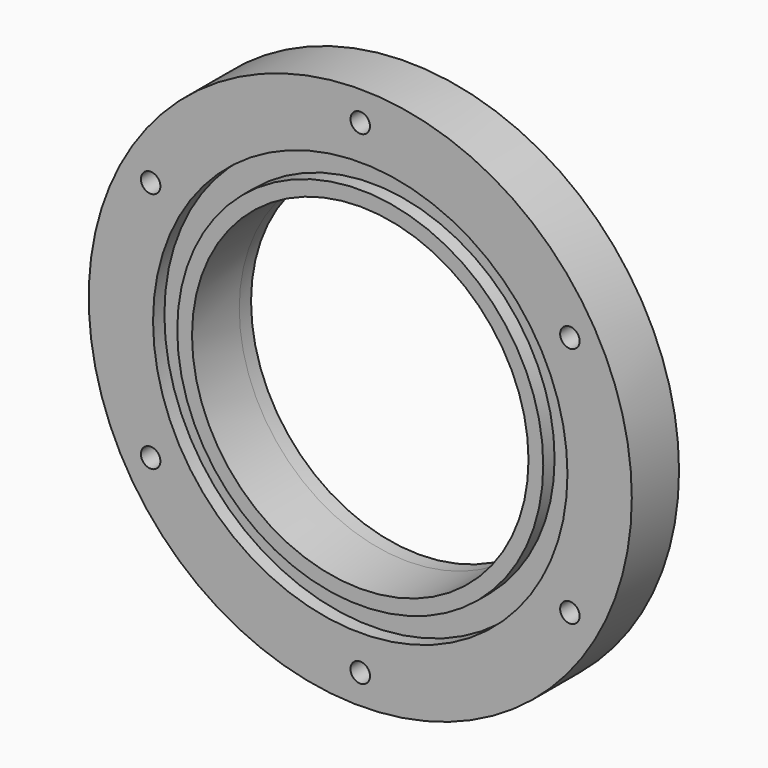
from build123d import *
from build123d import SkipClean  # not in build123d's __all__

# Parameters (mm, degrees)
F0_R     = 46
F0_R_2   = 28.5
F1_DEPTH = 10
F2_R     = 35.1
F2_R_2   = 31
F3_DEPTH = 2.4
F5_D     = 3.3
F5_DEPTH = 8
F5_TIP   = 0.9914200214
F6_R     = 30.5
F6_R_2   = 28.5
F7_DEPTH = 2.5


with BuildPart() as f1:
    # F0 (on Front) → F1 (new body)
    with BuildSketch(Plane.XZ):
        Circle(F0_R)
        Circle(F0_R_2, mode=Mode.SUBTRACT)
    extrude(amount=-F1_DEPTH)

    # F2 (on face) → F3 (cut)
    with BuildSketch(Plane.XZ):
        Circle(F2_R)
        Circle(F2_R_2, mode=Mode.SUBTRACT)
    extrude(amount=-F3_DEPTH, mode=Mode.SUBTRACT)

    # F5
    with Locations(Plane.XZ):
        with Locations((0, 41), (35.5070415552, 20.5), (35.5070415552, -20.5), (0, -41), (-35.5070415552, -20.5), (-35.5070415552, 20.5)):
            Hole(F5_D / 2, depth=F5_DEPTH)
            with Locations((0, 0, -(F5_DEPTH + F5_TIP / 2))):  # 118° drill point
                Cone(0, F5_D / 2, F5_TIP, mode=Mode.SUBTRACT)

    # F6 (on face) → F7 (join)
    with BuildSketch(Plane(origin=(0, 10, 0), x_dir=(-1, 0, 0), z_dir=(0, 1, 0))):
        Circle(F6_R)
        Circle(F6_R_2, mode=Mode.SUBTRACT)
    with SkipClean():  # cleaning this boolean's faces spoils the solid; the shape is the same uncleaned
        extrude(amount=F7_DEPTH)


solid = f1.part
